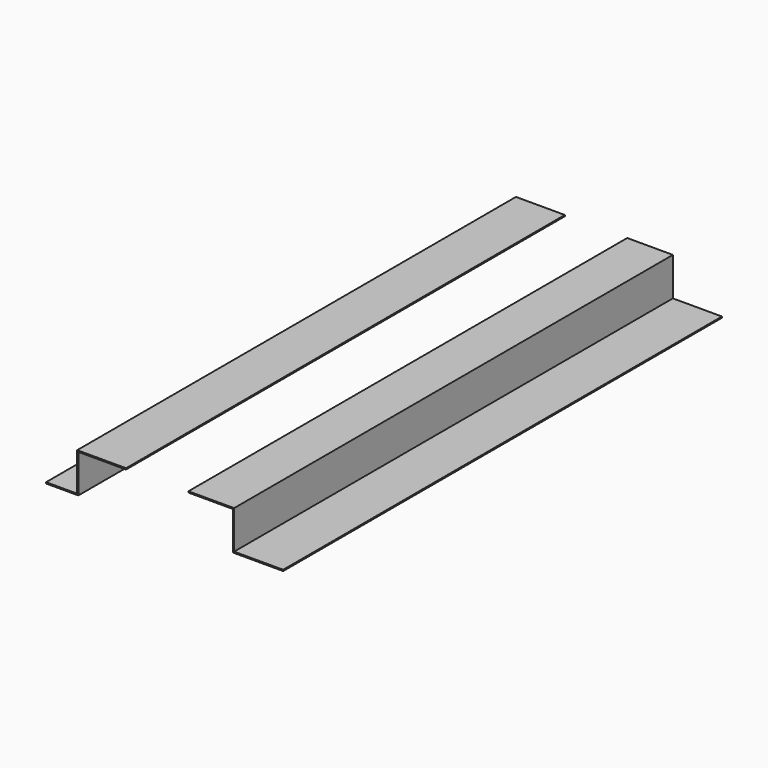
from build123d import *

# Parameters (mm, degrees)
F1_DEPTH = 917
F3_DEPTH = 2


# Not quite as in the source:
# - a feature names something its author has since deleted; it is built from what else it names


with BuildPart() as f1:
    # F0 (on Front) → F1 (new body)
    with BuildSketch(Plane.XZ):
        Polygon((133.3621336615, -66.0460090514), (211.4915523357, -66.0460090514), (211.4915523357, -64.0460090514), (129.4915523357, -64.0460090514), (129.4915523357, 0), (-132.8778128425, 0), (-132.8778128425, -64.0460090514), (-184.8778128425, -64.0460090514), (-184.8778128425, -66.0460090514), (-133.3621336615, -66.0460090514), (-130.8778128425, -66.0460090514), (-130.8778128425, -2), (127.4915523357, -2), (127.4915523357, -66.0460090514), align=None)
    extrude(amount=F1_DEPTH)

    # F2 (on Top) → F3 (cut)
    with BuildSketch(Plane.XY):
        Polygon((53.1499173463, 0), (-51.1629678309, 0), (-51.1629678309, -190.4399693012), (-51.1629678309, -198.6912098614), (-51.1629678309, -718.3087901386), (-51.1629678309, -917), (53.1499173463, -917), (53.1499173463, -718.3087901386), (53.1499173463, -198.6912098614), align=None)
    extrude(amount=-F3_DEPTH, mode=Mode.SUBTRACT)


solid = f1.part
